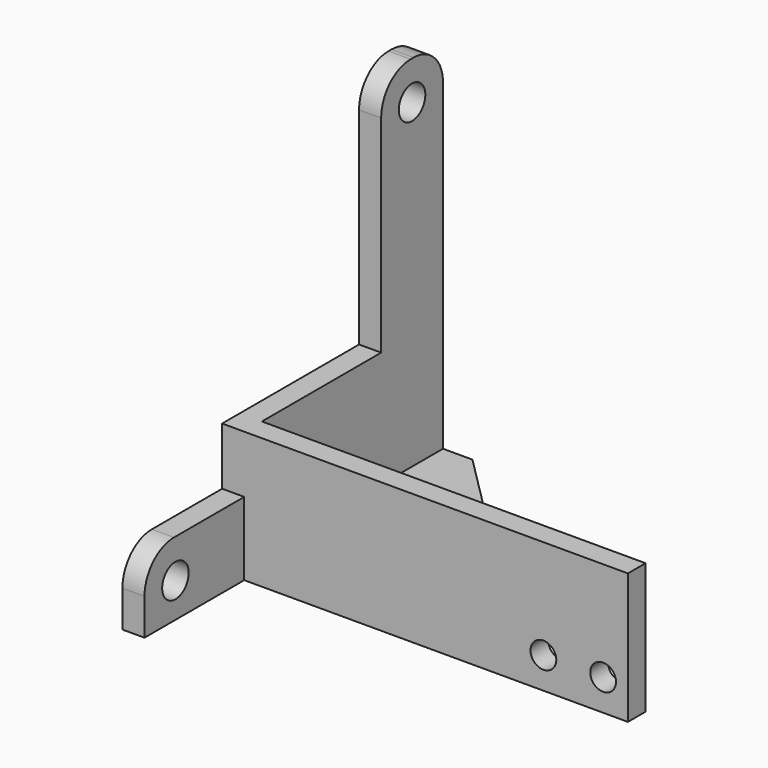
from build123d import *

# Parameters (mm, degrees)
F0_W        = 15.12
F0_H        = 17.76
F0_R        = 1.75
F0_W_2      = 3
F0_H_2      = 15.76
F0_W_3      = 35
F0_H_3      = 2
F1_DEPTH    = 3
F2_DEPTH    = 30.75
F4_DEPTH    = 3
F5_T4_DEPTH = 161.4443452539


# Not quite as in the source:
# - a fillet or chamfer that OpenCascade refuses, or shapes differently, is made with other operations: its cross-section is extruded or revolved along the edge and cut away or added


with BuildPart() as f1:
    # F0 (on Front) → F1 (new body)
    with BuildSketch(Plane.XZ):
        Rectangle(F0_W, F0_H)
        with Locations((-3.9189920692, -4.63)):
            Circle(F0_R, mode=Mode.SUBTRACT)
        with Locations((4.1910079308, -4.63)):
            Circle(F0_R, mode=Mode.SUBTRACT)
        Polygon((-7.56, -8.88), (-7.56, 8.88), (-44.56, 8.88), (-44.56, -6.88), (-9.56, -6.88), (-9.56, -8.88), align=None)
        with Locations((-46.06, 1)):
            Rectangle(F0_W_2, F0_H_2)
        with Locations((-27.06, -7.88)):
            Rectangle(F0_W_3, F0_H_3)
        with Locations((-46.06, -7.88)):
            Rectangle(F0_W_2, F0_H_3)
    extrude(amount=F1_DEPTH)

    # F0 (on Front) → F2 (join)
    with BuildSketch(Plane.XZ):
        with Locations((-46.06, 1)):
            Rectangle(F0_W_2, F0_H_2)
        with Locations((-46.06, -7.88)):
            Rectangle(F0_W_2, F0_H_3)
        with Locations((-27.06, -7.88)):
            Rectangle(F0_W_3, F0_H_3)
    extrude(amount=-F2_DEPTH)

    # F3 (on face) → F4 (join)
    with BuildSketch(Plane(origin=(-47.56, 0, 0), x_dir=(0, -1, 0), z_dir=(-1, 0, 0))):
        with BuildLine():
            Line((-30.75, 36.9310820997), (-30.75, 34.42))
            Line((-30.75, 34.42), (-23.2759684913, 34.42))
            Line((-23.2759684913, 34.42), (-20.25, 34.42))
            Line((-20.25, 34.42), (-20.25, 36.9310820997))
            ThreePointArc((-20.25, 36.9310820997), (-21.7144660941, 40.4666160056), (-25.25, 41.9310820997))
            Line((-25.25, 41.9310820997), (-25.75, 41.9310820997))
            ThreePointArc((-25.75, 41.9310820997), (-29.2855339059, 40.4666160056), (-30.75, 36.9310820997))
        make_face()
        with BuildLine():
            Line((-23.2759684913, 36.3402245806), (-23.2759684913, 34.42))
            Line((-23.2759684913, 34.42), (-23.922206416, 35.0770037331))
            ThreePointArc((-23.922206416, 35.0770037331), (-27.6352195224, 37.3905449889), (-23.2759684913, 37.0219396188))
            ThreePointArc((-23.2759684913, 37.0219396188), (-23.2565015161, 36.852004751), (-23.25, 36.6810820997))
            ThreePointArc((-23.25, 36.6810820997), (-23.2565015161, 36.5101594484), (-23.2759684913, 36.3402245806))
        make_face(mode=Mode.SUBTRACT)
        Polygon((-30.75, 34.42), (-30.75, 8.88), (-20.25, 8.88), (-20.25, 31.3436212872), (-23.2759684913, 34.42), align=None)
        Polygon((-23.2759684913, 34.42), (-20.25, 31.3436212872), (-20.25, 34.42), align=None)
        with BuildLine():
            Line((3, 1.0805530297), (3, -8.88))
            Line((3, -8.88), (19.3145081394, -8.88))
            Line((19.3145081394, -8.88), (16.2589368567, -5.7735253369))
            ThreePointArc((16.2589368567, -5.7735253369), (13.0770649061, -5.7472405543), (13.1033496887, -2.5653686037))
            Line((13.1033496887, -2.5653686037), (9.517170933, 1.0805530297))
            Line((9.517170933, 1.0805530297), (3, 1.0805530297))
        make_face()
        with BuildLine():
            Line((16.2589368567, -5.7735253369), (19.3145081394, -8.88))
            Line((19.3145081394, -8.88), (19.9311432727, -8.88))
            Line((19.9311432727, -8.88), (19.9311432727, -3.9194469703))
            ThreePointArc((19.9311432727, -3.9194469703), (18.4666771787, -0.3839130644), (14.9311432727, 1.0805530297))
            Line((14.9311432727, 1.0805530297), (9.517170933, 1.0805530297))
            Line((9.517170933, 1.0805530297), (13.1033496887, -2.5653686037))
            ThreePointArc((13.1033496887, -2.5653686037), (15.5507594053, -2.0942920889), (16.9311432727, -4.1694469703))
            ThreePointArc((16.9311432727, -4.1694469703), (16.7562981542, -5.0390631029), (16.2589368567, -5.7735253369))
        make_face()
        with BuildLine():
            Line((-23.922206416, 35.0770037331), (-23.2759684913, 34.42))
            Line((-23.2759684913, 34.42), (-23.2759684913, 36.3402245806))
            ThreePointArc((-23.2759684913, 36.3402245806), (-23.4969023398, 35.6563383445), (-23.922206416, 35.0770037331))
        make_face()
    extrude(amount=-F4_DEPTH)

    # F5: chamfer of 31 on 1 edges, made by hand


with BuildPart() as f5_tool2:
    # F5_s3 → F5_t4 (new body)
    with BuildSketch(Plane.XY.offset(-88.6021726269)):
        Polygon((-9.56, -0.25), (-40.56, 30.75), (-9.56, 30.75), align=None)
    extrude(amount=F5_T4_DEPTH)

    split(bisect_by=Plane.XZ, keep=Keep.BOTTOM)


with BuildPart() as f1_1:
    add(f1.part)

    # F5_t1: cut F5_tool2
    add(f5_tool2.part, mode=Mode.SUBTRACT)


solid = f1_1.part
